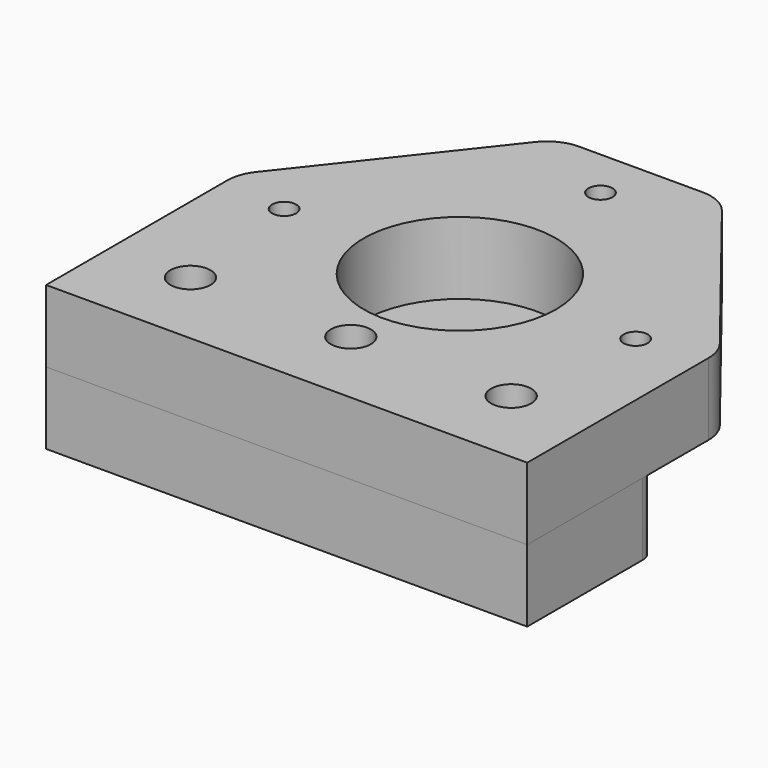
from build123d import *

# Parameters (mm, degrees)
F0_R     = 2.5
F0_R_2   = 1.5
F0_R_3   = 12
F2_DEPTH = 9
F1_R     = 2.5
F1_R_2   = 12
F3_DEPTH = 9
F1_R_3   = 4.5
F4_DEPTH = 5


with BuildPart() as f2:
    # F0 (on Top) → F2 (new body)
    with BuildSketch(Plane.XY):
        with BuildLine():
            Line((-1.4435148332, 28.2101202756), (-7.7092999779, 28.2101202756))
            ThreePointArc((-7.7092999779, 28.2101202756), (-9.8918540281, 27.7086153371), (-11.6365834243, 26.3047034029))
            Line((-11.6365834243, 26.3047034029), (-28.9272834464, 4.3613665526))
            ThreePointArc((-28.9272834464, 4.3613665526), (-29.7242151323, 2.9044010192), (-30, 1.2667834253))
            Line((-30, 1.2667834253), (-30, 0))
            Line((-30, 0), (-30, -27))
            Line((-30, -27), (30, -27))
            Line((30, -27), (30, 0))
            Line((30, 0), (30, 1.2667834253))
            ThreePointArc((30, 1.2667834253), (29.7242151323, 2.9044010192), (28.9272834464, 4.3613665526))
            Line((28.9272834464, 4.3613665526), (11.6365834243, 26.3047034029))
            ThreePointArc((11.6365834243, 26.3047034029), (9.8918540281, 27.7086153371), (7.7092999779, 28.2101202756))
            Line((7.7092999779, 28.2101202756), (-1.4435148332, 28.2101202756))
        make_face()
        with Locations((-20, -17)):
            Circle(F0_R, mode=Mode.SUBTRACT)
        with Locations((-21.9206204292, 0)):
            Circle(F0_R_2, mode=Mode.SUBTRACT)
        with Locations((0, -17)):
            Circle(F0_R, mode=Mode.SUBTRACT)
        with Locations((20, -17)):
            Circle(F0_R, mode=Mode.SUBTRACT)
        Circle(F0_R_3, mode=Mode.SUBTRACT)
        with Locations((21.9206204292, 0)):
            Circle(F0_R_2, mode=Mode.SUBTRACT)
        with Locations((0, 21.92)):
            Circle(F0_R_2, mode=Mode.SUBTRACT)
    extrude(amount=F2_DEPTH)


with BuildPart() as f3:
    # F1 (on Top) → F3 (new body)
    with BuildSketch(Plane.XY):
        with BuildLine():
            ThreePointArc((-28, -7), (-29.4142135624, -7.5857864376), (-30, -9))
            Line((-30, -9), (-30, -27))
            Line((-30, -27), (30, -27))
            Line((30, -27), (30, -9))
            ThreePointArc((30, -9), (29.4142135624, -7.5857864376), (28, -7))
            Line((28, -7), (17, -7))
            ThreePointArc((17, -7), (15.5857864376, -6.4142135624), (15, -5))
            Line((15, -5), (15, -0.3713906764))
            ThreePointArc((15, -0.3713906764), (14.9663841605, -0.0062423047), (14.8666666667, 0.3466312979))
            Line((14.8666666667, 0.3466312979), (10.1079539748, 12.7180219743))
            ThreePointArc((10.1079539748, 12.7180219743), (9.3735319927, 13.6486424641), (8.2412873082, 14))
            Line((8.2412873082, 14), (0, 14))
            Line((0, 14), (-8.2412873082, 14))
            ThreePointArc((-8.2412873082, 14), (-9.3735319927, 13.6486424641), (-10.1079539748, 12.7180219743))
            Line((-10.1079539748, 12.7180219743), (-14.8666666667, 0.3466312979))
            ThreePointArc((-14.8666666667, 0.3466312979), (-14.9663841605, -0.0062423047), (-15, -0.3713906764))
            Line((-15, -0.3713906764), (-15, -5))
            ThreePointArc((-15, -5), (-15.5857864376, -6.4142135624), (-17, -7))
            Line((-17, -7), (-28, -7))
        make_face()
        with Locations((-20, -17)):
            Circle(F1_R, mode=Mode.SUBTRACT)
        with Locations((0, -17)):
            Circle(F1_R, mode=Mode.SUBTRACT)
        with Locations((20, -17)):
            Circle(F1_R, mode=Mode.SUBTRACT)
        Circle(F1_R_2, mode=Mode.SUBTRACT)
    extrude(amount=-F3_DEPTH)

    # F1 (on Top) → F4 (join)
    with BuildSketch(Plane.XY):
        Circle(F1_R_2)
        Circle(F1_R_3, mode=Mode.SUBTRACT)
    extrude(amount=-F4_DEPTH)


solid = Compound([f2.part, f3.part])
